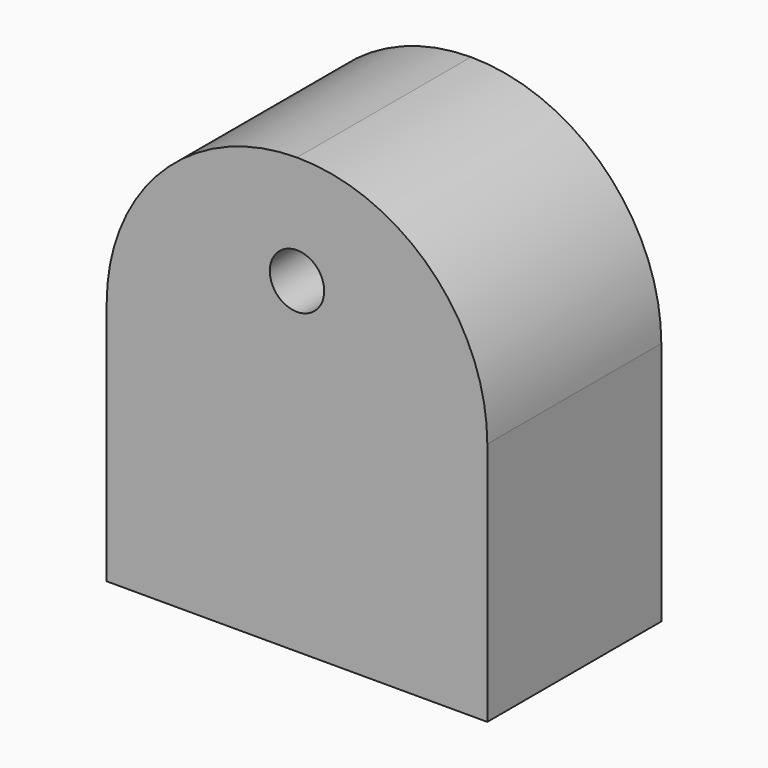
from build123d import *

# Parameters (mm, degrees)
F1_DEPTH = 40
F2_R     = 17.49999
F3_R     = 2.5
F4_DEPTH = 25
F5_R     = 1
F6_DEPTH = 25


# Not quite as in the source:
# - a fillet or chamfer is up to 0.001 mm smaller than in the source, because OpenCascade refuses the exact size


with BuildPart() as f1:
    # F0 (on Top) → F1 (new body)
    with BuildSketch(Plane.XY):
        Polygon((17.5, 10), (0, 10), (-17.5, 10), (-17.5, -10), (17.5, -10), align=None)
    extrude(amount=F1_DEPTH)

    # F2 (radius 17.5 in the source; OpenCascade refuses exactly that, so slightly less here)
    f2_edges = [f1.edges().sort_by_distance(p)[0] for p in [
        (17.5, 0, 40),
        (-17.5, 0, 40),
    ]]
    fillet(f2_edges, radius=F2_R)

    # F3 (on face) → F4 (cut)
    with BuildSketch(Plane.XZ.offset(10)):
        with Locations((0, 30)):
            Circle(F3_R)
    extrude(amount=-F4_DEPTH, mode=Mode.SUBTRACT)

    # F5 (on face) → F6 (cut)
    with BuildSketch(Plane(origin=(0, 0, 0), x_dir=(1, 0, 0), z_dir=(0, 0, -1))):
        with Locations((10, 0)):
            Circle(F5_R)
        with Locations((-10, 0)):
            Circle(F5_R)
    extrude(amount=-F6_DEPTH, mode=Mode.SUBTRACT)


solid = f1.part
